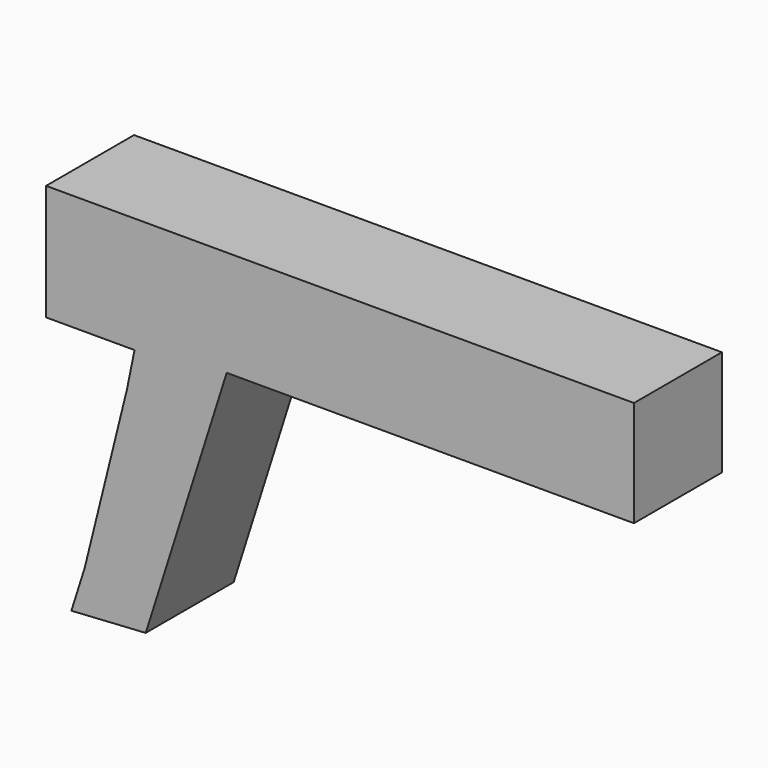
from build123d import *

# Parameters (mm, degrees)
F1_DEPTH = 25


# Not quite as in the source:
# - the program builds the solid bodies; features that only make, move or delete a surface that nothing else refers to are left out


with BuildPart() as f1:
    # F0 (on Front) → F1 (new body)
    with BuildSketch(Plane.XZ):
        Polygon((-64.7279694676, 8.3565656096), (-66.4276108146, 0), (-76.058909297, -38.9500930905), (-79.0885544769, -48.5051267807), (-62.1785111725, -47.4482923746), (-43.7657386065, 10.6227528304), (48.864658922, 10.6227528304), (48.864658922, 34.7009897232), (-84.8403796554, 34.7009897232), (-84.8403796554, 8.3565656096), align=None)
    extrude(amount=F1_DEPTH)


solid = f1.part
